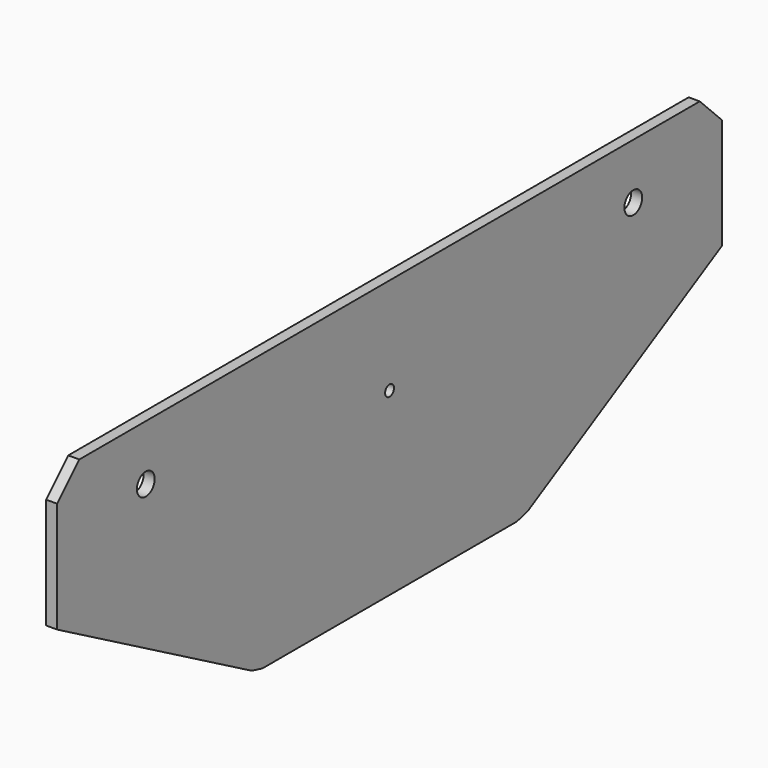
from build123d import *

# Parameters (mm, degrees)
F1_DEPTH    = 2
F3_D        = 8
F5_T1_DEPTH = 55.4336597593
F5_T3_DEPTH = 18.9008056118
F6_D        = 4


# Not quite as in the source:
# - a fillet or chamfer that OpenCascade refuses, or shapes differently, is made with other operations: its cross-section is extruded or revolved along the edge and cut away or added
# - a feature of the source that left no trace in its solid (it failed there, or was rolled back) is left out


with BuildPart() as f1:
    # F0 (on Right) → F1 (new body, symmetric)
    with BuildSketch(Plane.YZ):
        Polygon((150, 100), (-150, 100), (-150, 50), (-60, 0), (60, 0), (150, 50), align=None)
    extrude(amount=F1_DEPTH, both=True)

    # F3 (through all)
    with Locations(Plane.YZ.offset(2)):
        with Locations((-110, 80), (110, 80)):
            Hole(F3_D / 2)

    # F5: chamfer of 10 on 4 edges, made by hand

    # F5_s2 → F5_t1 (cut)
    with BuildSketch(Plane.YZ.offset(-27.7168298797)):
        Polygon((140, 100), (150, 90), (150, 100), align=None)
        Polygon((-140, 100), (-150, 90), (-150, 100), align=None)
    extrude(amount=F5_T1_DEPTH, mode=Mode.SUBTRACT)

    # F5_s4 → F5_t3 (cut)
    with BuildSketch(Plane.YZ.offset(-9.4504028059)):
        Polygon((-62.2651690298, 1.2584272388), (-57.408739718, 0), (-60, 0), align=None)
        Polygon((62.2651690298, 1.2584272388), (57.408739718, 0), (60, 0), align=None)
    extrude(amount=F5_T3_DEPTH, mode=Mode.SUBTRACT)

    # F6 (through all)
    with Locations(Plane.YZ.offset(2)):
        with Locations((0, 65)):
            Hole(F6_D / 2)


solid = f1.part
